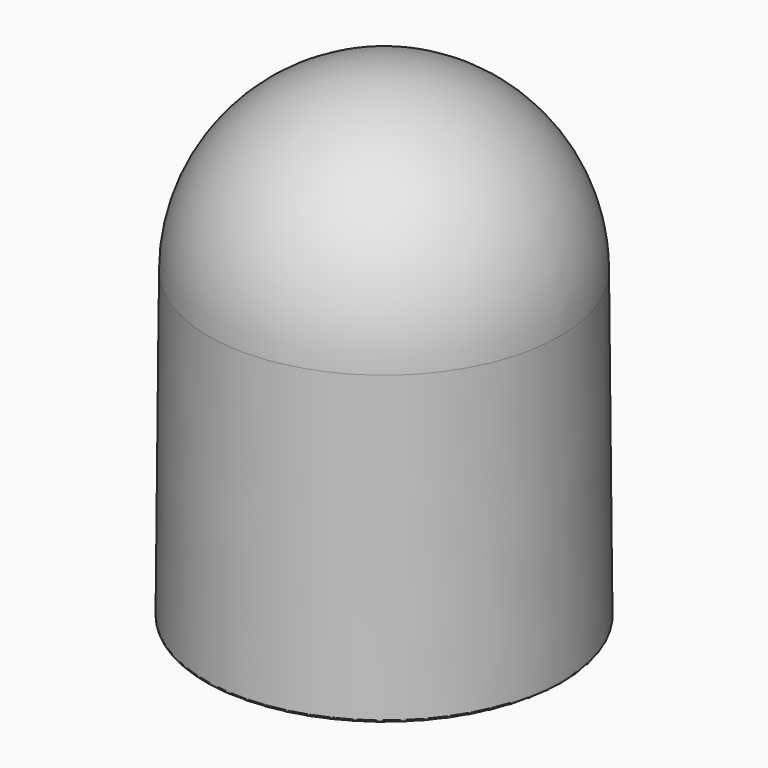
from build123d import *

# Parameters (mm, degrees)
F4_ANGLE        = 5
F4_COPIES_COUNT = 3


# Not quite as in the source:
# - a pattern or mirror of a feature is missing from the dataset's text; its kind, count and spacing are read off the source's solid
# - a feature names something its author has since deleted; it is built from what else it names


with BuildPart() as f1:
    # F0 (on Front) → F1 (revolve)
    with BuildSketch(Plane.XZ):
        with BuildLine():
            Line((19.3359252066, -32.76378346), (19.05, 0))
            ThreePointArc((19.05, 0), (13.4703841816, 13.4703841816), (0, 19.05))
            Line((0, 19.05), (0, 17.78))
            ThreePointArc((0, 17.78), (3.7797166534, 17.3736047503), (7.3866482795, 16.1729968526))
            ThreePointArc((7.3866482795, 16.1729968526), (7.4718390154, 16.1273495327), (7.5505663952, 16.071285828))
            Line((7.5505663952, 16.071285828), (11.0474861959, 13.9014506367))
            ThreePointArc((11.0474861959, 13.9014506367), (11.1326769319, 13.8558033168), (11.2114043116, 13.7997396121))
            ThreePointArc((11.2114043116, 13.7997396121), (16.0540831046, 7.641650062), (17.78, 0))
            Line((17.78, 0), (18.0570780524, -31.75))
            Line((18.0570780524, -31.75), (18.0570780524, -32.131))
            ThreePointArc((18.0570780524, -32.131), (18.3174601239, -32.7596179285), (18.9460780524, -33.02))
            Line((18.9460780524, -33.02), (19.0819348781, -33.02))
            ThreePointArc((19.0819348781, -33.02), (19.2623219635, -32.94481974), (19.3359252066, -32.76378346))
        make_face()
    revolve(axis=Axis((0, 0, -9.9657937262), (0, 0, -1)))

    # F0 (on Front) → F2 (revolve)
    with BuildSketch(Plane.XZ):
        with BuildLine():
            Line((11.0474861959, 13.9014506367), (7.5505663952, 16.071285828))
            ThreePointArc((7.5505663952, 16.071285828), (7.7566742417, 15.8103666839), (7.8320486243, 15.4865180361))
            Line((7.8320486243, 15.4865180361), (7.9671974198, 0))
            Line((7.9671974198, 0), (8.0429513757, -8.6805435522))
            ThreePointArc((8.0429513757, -8.6805435522), (8.268463141, -9.2150551884), (8.8049223611, -9.4358939321))
            Line((8.8049223611, -9.4358939321), (9.3967179228, -9.4358939321))
            ThreePointArc((9.3967179228, -9.4358939321), (9.5228386444, -9.3842965826), (9.5766292455, -9.2590955677))
            Line((9.5766292455, -9.2590955677), (9.9690316117, 13.2216209339))
            ThreePointArc((9.9690316117, 13.2216209339), (10.3245683016, 13.852935192), (11.0474861959, 13.9014506367))
        make_face()
    revolve(axis=Axis((0, 0, -9.9657937262), (0, 0, -1)))

    # F3 (on Front) → F4 (revolve, cut)
    with BuildSketch(Plane.XZ):
        with BuildLine():
            Line((7.9002389035, 7.6726859874), (8.0429513757, -8.6805435522))
            ThreePointArc((8.0429513757, -8.6805435522), (8.268463141, -9.2150551884), (8.8049223611, -9.4358939321))
            Line((8.8049223611, -9.4358939321), (9.3967179228, -9.4358939321))
            ThreePointArc((9.3967179228, -9.4358939321), (9.5228386444, -9.3842965826), (9.5766292455, -9.2590955677))
            Line((9.5766292455, -9.2590955677), (9.8724750188, 7.6898974312))
            Line((9.8724750188, 7.6898974312), (7.9002389035, 7.6726859874))
        make_face()
    f4 = revolve(axis=Axis((0, 0, -9.9657937262), (0, 0, 1)), revolution_arc=F4_ANGLE, mode=Mode.SUBTRACT)

    # F4_copies: F4 ×3 about axis
    f4_copies_axis = Axis((0, 0, 0), (0, 0, 1))
    for i in range(1, F4_COPIES_COUNT):
        add(f4.rotate(f4_copies_axis, i * 360 / F4_COPIES_COUNT), mode=Mode.SUBTRACT)


solid = f1.part
